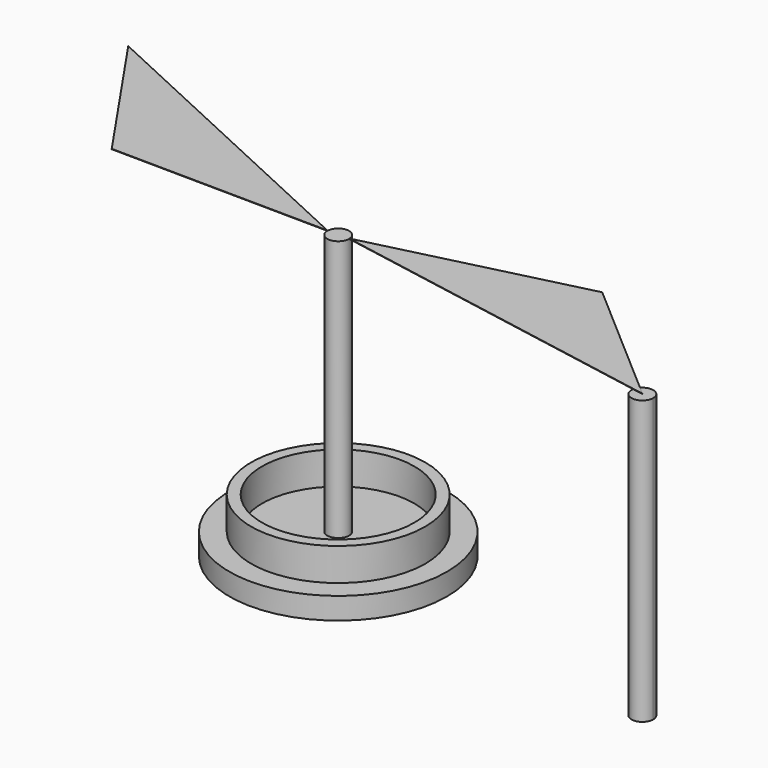
from build123d import *

# Parameters (mm, degrees)
F0_R      = 63.5
F1_DEPTH  = 12.7
F2_R      = 50.8
F2_R_2    = 44.45
F3_DEPTH  = 31.75
F4_R      = 6.35
F5_DEPTH  = 152.4
F7_DEPTH  = 0.254
F9_DEPTH  = 0.254
F13_DEPTH = 165.1


# Not quite as in the source:
# - the program builds the solid bodies; features that only make, move or delete a surface that nothing else refers to are left out


with BuildPart() as f1:
    # F0 (on Top) → F1 (new body)
    with BuildSketch(Plane.XY):
        Circle(F0_R)
    extrude(amount=F1_DEPTH)

    # F2 (on Top) → F3 (join)
    with BuildSketch(Plane.XY):
        Circle(F2_R)
        Circle(F2_R_2, mode=Mode.SUBTRACT)
    extrude(amount=F3_DEPTH)

    # F4 (on face) → F5 (join)
    with BuildSketch(Plane.XY.offset(12.7)):
        Circle(F4_R)
    extrude(amount=F5_DEPTH)


with BuildPart() as f7:
    # F6 (on face) → F7 (new body)
    with BuildSketch(Plane.XY.offset(165.1)):
        Polygon((129.6198948271, 30.5537727509), (6.35, 0), (206.3221851049, -36.0744394879), align=None)
    extrude(amount=F7_DEPTH)


with BuildPart() as f9:
    # F8 (on face) → F9 (new body)
    with BuildSketch(Plane.XY.offset(165.1)):
        Polygon((-133.3409966481, 1.5122071029), (-6.35, 0), (-190.7670811897, 85.3263157853), align=None)
    extrude(amount=F9_DEPTH)


with BuildPart() as f13:
    # F12 (on face) → F13 (new body)
    with BuildSketch(Plane(origin=(0, 0, 165.1), x_dir=(1, 0, 0), z_dir=(0, 0, -1))):
        with BuildLine():
            ThreePointArc((201.5282919625, 31.910176223), (208.5449399886, 30.1261741335), (212.6721851049, 36.0744394879))
            ThreePointArc((212.6721851049, 36.0744394879), (205.7562701297, 42.3991719124), (200.0730543204, 34.9471132539))
            Line((200.0730543204, 34.9471132539), (206.3221851049, 36.0744394879))
            Line((206.3221851049, 36.0744394879), (201.5282919625, 31.910176223))
        make_face()
    extrude(amount=F13_DEPTH)


solid = Compound([f1.part, f7.part, f9.part, f13.part])
